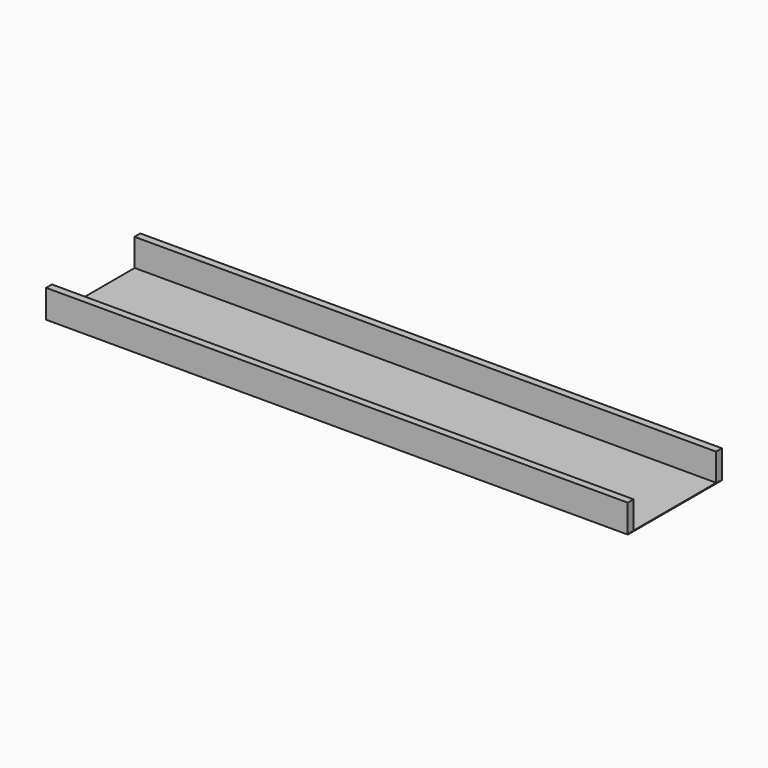
from build123d import *

# Parameters (mm, degrees)
F1_W     = 200.1392990351
F1_H     = 2.5080107152
F2_DEPTH = 9.6774
F0_W     = 200.1125812531
F0_H     = 40.237609297
F3_DEPTH = 0.254


# Not quite as in the source:
# - a feature names something its author has since deleted; it is built from what else it names


with BuildPart() as f2:
    # F1 (on Top) → F2 (new body)
    with BuildSketch(Plane.XY):
        with Locations((-0.0575333834, 19.0099850297)):
            Rectangle(F1_W, F1_H)
    extrude(amount=F2_DEPTH)


with BuildPart() as f3:
    # F0 (on Top) → F3 (new body)
    with BuildSketch(Plane.XY):
        Rectangle(F0_W, F0_H)
    extrude(amount=F3_DEPTH)


with BuildPart() as f4_1:
    # F4: instance of F2
    add(f2.part.mirror(Plane.XZ))


solid = Compound([f2.part, f3.part, f4_1.part])
